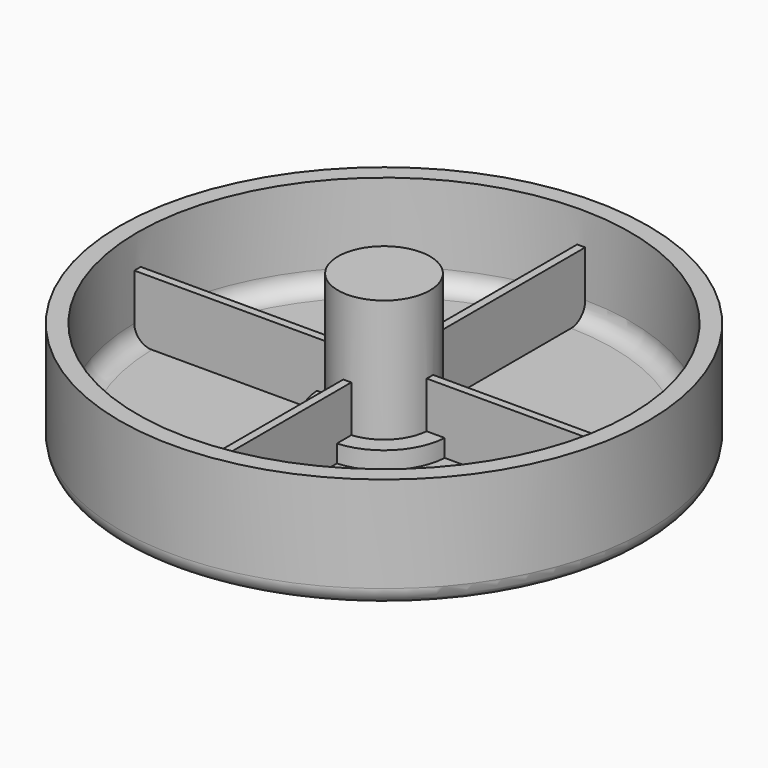
from build123d import *

# Parameters (mm, degrees)
F0_R            = 33
F1_DEPTH        = 2.2
F2_R            = 33
F2_R_2          = 30.8
F3_DEPTH        = 12
F4_R            = 2.2
F5_R            = 2.2
F6_R            = 8
F7_DEPTH        = 2.2
F8_R            = 5.75
F9_DEPTH        = 15.3
F10_W           = 1
F10_H           = 63
F11_DEPTH       = 8
F12_W           = 63
F12_H           = 1
F13_DEPTH       = 8
F15_D           = 0.01
F15_DEPTH       = 2.4
F15_CBORE_D     = 12.2
F15_CBORE_DEPTH = 2.4
F15_TIP         = 0.0030043031


with BuildPart() as f1:
    # F0 (on Top) → F1 (new body)
    with BuildSketch(Plane.XY):
        Circle(F0_R)
    extrude(amount=F1_DEPTH)

    # F2 (on face) → F3 (join)
    with BuildSketch(Plane.XY.offset(2.2)):
        Circle(F2_R)
        Circle(F2_R_2, mode=Mode.SUBTRACT)
    extrude(amount=F3_DEPTH)

    # F4
    f4_edges = [f1.edges().sort_by_distance(p)[0] for p in [
        (-33, 0, 0),
    ]]
    fillet(f4_edges, radius=F4_R)

    # F5
    f5_edges = [f1.edges().sort_by_distance(p)[0] for p in [
        (-30.8, 0, 2.2),
    ]]
    fillet(f5_edges, radius=F5_R)

    # F6 (on face) → F7 (join)
    with BuildSketch(Plane.XY.offset(2.2)):
        Circle(F6_R)
    extrude(amount=F7_DEPTH)

    # F8 (on face) → F9 (join)
    with BuildSketch(Plane.XY.offset(4.4)):
        Circle(F8_R)
    extrude(amount=F9_DEPTH)

    # F10 (on face) → F11 (join)
    with BuildSketch(Plane.XY.offset(2.2)):
        Rectangle(F10_W, F10_H)
    extrude(amount=F11_DEPTH)

    # F12 (on face) → F13 (join)
    with BuildSketch(Plane.XY.offset(2.2)):
        Rectangle(F12_W, F12_H)
    extrude(amount=F13_DEPTH)

    # F15
    with Locations(Plane(origin=(0, 0, 0), x_dir=(1, 0, 0), z_dir=(0, 0, -1))):
        with Locations((0, 0)):
            CounterBoreHole(F15_D / 2, F15_CBORE_D / 2, F15_CBORE_DEPTH, depth=F15_DEPTH)
            with Locations((0, 0, -(F15_DEPTH + F15_TIP / 2))):  # 118° drill point
                Cone(0, F15_D / 2, F15_TIP, mode=Mode.SUBTRACT)


solid = f1.part
